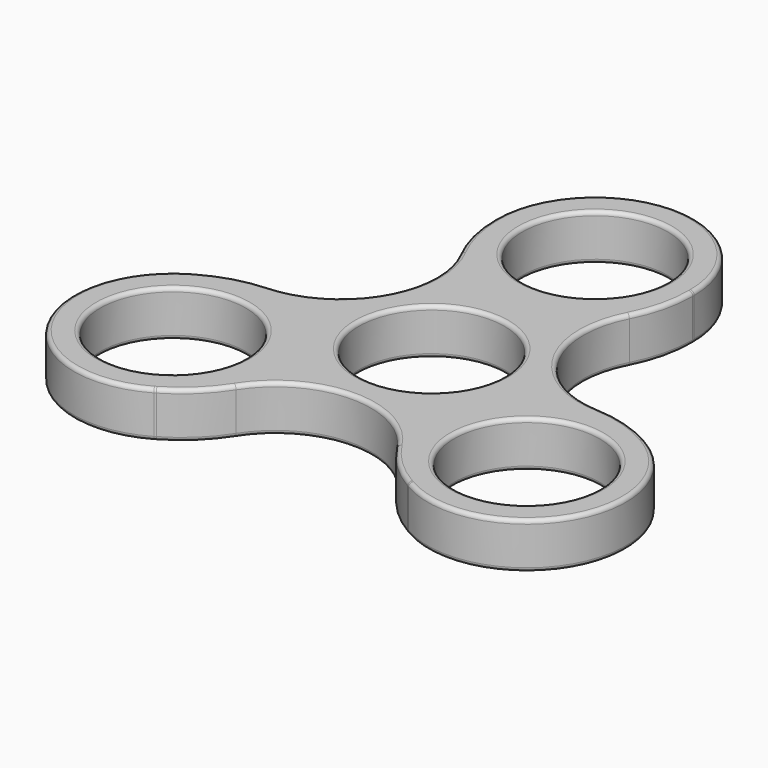
from build123d import *

# Parameters (mm, degrees)
F0_R            = 15.05
F0_R_2          = 11.05
F1_DEPTH        = 7
F2_R            = 11.05
F3_DEPTH        = 7
F3_COPIES_COUNT = 3
F5_DEPTH        = 118
F5_COPIES_COUNT = 3
F6_R            = 20
F7_R            = 0.6


# Not quite as in the source:
# - an extrude ends at something that could not be found from the text; its depth is read off the source's solid
# - a pattern or mirror of a feature is missing from the dataset's text; its kind, count and spacing are read off the source's solid


with BuildPart() as f1:
    # F0 (on Top) → F1 (new body)
    with BuildSketch(Plane.XY):
        Circle(F0_R)
        Circle(F0_R_2, mode=Mode.SUBTRACT)
    extrude(amount=F1_DEPTH)

    # F2 (on Top) → F3 (join, through all)
    with BuildSketch(Plane.XY):
        with BuildLine():
            Line((15.05, 0), (15.05, 31))
            ThreePointArc((15.05, 31), (0, 46.05), (-15.05, 31))
            Line((-15.05, 31), (-15.05, 0))
            ThreePointArc((-15.05, 0), (0, 15.05), (15.05, 0))
        make_face()
        with Locations((0, 31)):
            Circle(F2_R, mode=Mode.SUBTRACT)
    f3 = extrude(amount=F3_DEPTH)

    # F3_copies: F3 ×3 about axis
    f3_copies_axis = Axis((0, 0, 0), (0, 0, 1))
    for i in range(1, F3_COPIES_COUNT):
        add(f3.rotate(f3_copies_axis, i * 360 / F3_COPIES_COUNT))

    # F4 (on Top) → F5 (cut, through all)
    with BuildSketch(Plane.XY):
        with BuildLine():
            Line((15.05, 8.6891215513), (15.05, 24.6891215513))
            ThreePointArc((15.05, 24.6891215513), (13.1204970221, 7.5751224876), (28.9064064606, 0.6891215513))
            Line((28.9064064606, 0.6891215513), (15.05, 8.6891215513))
        make_face()
    f5 = extrude(amount=F5_DEPTH, mode=Mode.SUBTRACT)

    # F5_copies: F5 ×3 about axis
    f5_copies_axis = Axis((0, 0, 0), (0, 0, 1))
    for i in range(1, F5_COPIES_COUNT):
        add(f5.rotate(f5_copies_axis, i * 360 / F5_COPIES_COUNT), mode=Mode.SUBTRACT)

    # F6
    f6_edges = [f1.edges().sort_by_distance(p)[0] for p in [
        (15.05, 24.689122, 3.5),
        (28.906406, 0.689122, 3.5),
        (13.856406, -25.378243, 3.5),
        (-13.856406, -25.378243, 3.5),
        (-28.906406, 0.689122, 3.5),
        (-15.05, 24.689122, 3.5),
    ]]
    fillet(f6_edges, radius=F6_R)

    # F7
    f7_edges = [f1.edges().sort_by_distance(p)[0] for p in [
        (-11.05, 31, 7),
        (-11.05, 0, 7),
        (-11.05, 0, 0),
        (-11.05, 31, 0),
        (34.244231, -2.392673, 7),
        (29.728941, -0.443118, 7),
        (39.88047, -23.025, 7),
        (13.120497, 7.575122, 7),
        (19.194231, -28.460037, 7),
        (14.480719, 25.967577, 7),
        (15.248222, -25.524459, 7),
        (15.05, 30.85271, 7),
        (0, -15.150245, 7),
        (0, 46.05, 7),
        (-15.248222, -25.524459, 7),
        (-15.05, 30.85271, 7),
        (-19.194231, -28.460037, 7),
        (-14.480719, 25.967577, 7),
        (-39.88047, -23.025, 7),
        (-13.120497, 7.575122, 7),
        (-34.244231, -2.392673, 7),
        (-29.728941, -0.443118, 7),
        (-21.321788, -25.069581, 7),
        (32.371788, -5.930419, 7),
        (34.244231, -2.392673, 0),
        (29.728941, -0.443118, 0),
        (39.88047, -23.025, 0),
        (13.120497, 7.575122, 0),
        (19.194231, -28.460037, 0),
        (14.480719, 25.967577, 0),
        (15.248222, -25.524459, 0),
        (15.05, 30.85271, 0),
        (0, -15.150245, 0),
        (0, 46.05, 0),
        (-15.248222, -25.524459, 0),
        (-15.05, 30.85271, 0),
        (-19.194231, -28.460037, 0),
        (-14.480719, 25.967577, 0),
        (-39.88047, -23.025, 0),
        (-13.120497, 7.575122, 0),
        (-34.244231, -2.392673, 0),
        (-29.728941, -0.443118, 0),
        (-21.321788, -25.069581, 0),
        (32.371788, -5.930419, 0),
    ]]
    fillet(f7_edges, radius=F7_R)


solid = f1.part
